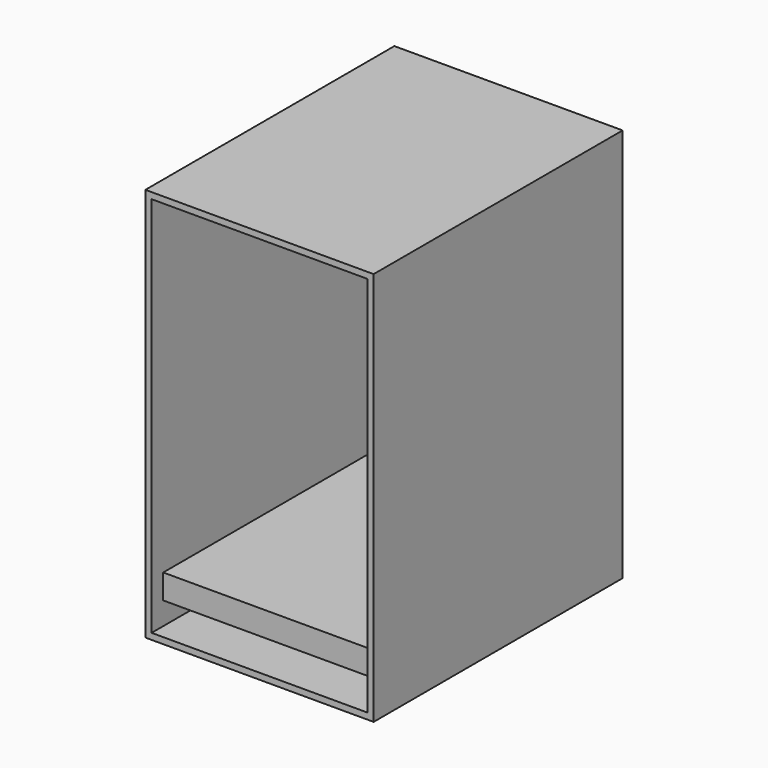
from build123d import *

# Parameters (mm, degrees)
F0_W         = 279.4
F0_H         = 482.6
F1_DEPTH     = 381
F2_T         = -7.62
F3_W         = 264.16
F3_H         = 30.1203280687
F4_DEPTH     = 355.6
F5_W         = 102.4026331621
F5_H         = 105.4210998118
F6_DEPTH     = 177.8
F7_DEPTH     = 177.8
F8_T         = 7.62
F8_T3_DEPTH  = 388.62
F8_T5_DEPTH  = 42.9501895142
F8_T7_DEPTH  = 370.84
F8_T9_DEPTH  = 45.3603280687
F8_T11_DEPTH = 146.3519571328
F8_T13_DEPTH = 193.04
F8_T15_DEPTH = 188.2364254725
F8_T17_DEPTH = 279.4
F8_T19_DEPTH = 424.7694824171
F8_T21_DEPTH = 117.6426331621
F8_T23_DEPTH = 120.6610998118


# Not quite as in the source:
# - a shell that OpenCascade refuses in one call is made with other operations: the cavity is built on its own and cut out


with BuildPart() as f1:
    # F0 (on Front) → F1 (new body)
    with BuildSketch(Plane.XZ):
        Rectangle(F0_W, F0_H)
    extrude(amount=F1_DEPTH)

    # F2
    f2_openings = [f1.faces().sort_by_distance(p)[0] for p in [
        (0, -381, 0),
    ]]
    offset(amount=F2_T, openings=f2_openings)

    # F3 (on face) → F4 (join)
    with BuildSketch(Plane.XZ.offset(7.62)):
        with Locations((0, -190.9096464515)):
            Rectangle(F3_W, F3_H)
    extrude(amount=F4_DEPTH)

    # F5 (on face) → F6 (join)
    with BuildSketch(Plane.XZ.offset(7.62)):
        with Locations((80.8786834189, 7.9730246216)):
            Rectangle(F5_W, F5_H)
    extrude(amount=F6_DEPTH)

    # F7 (add): a face of the model
    f7_faces = [f1.faces().sort_by_distance(p)[0] for p in [
        (80.8786834189, -185.42, 7.9730246216),
    ]]
    extrude(f7_faces, amount=-F7_DEPTH)

    # F8: shell of thickness 7.62, made by hand


with BuildPart() as f8_core1:
    # F8_t2: copy of F1
    add(f1.part)

    # the walls: a layer under each face that stays
    f8_faces = [f8_core1.faces().sort_by_distance(p)[0] for p in [
        (139.7, -190.5, 0),
        (0, -190.5, -241.3),
        (0, -190.5, 241.3),
        (0, 0, 0),
        (96.04375, -381, -235.3419753086),
        (-139.7, -190.5, 0),
        (132.08, -194.31, 0),
        (0, -194.31, -233.68),
        (-132.08, -194.31, 0),
        (0, -194.31, 233.68),
        (0, -7.62, -219.8249052429),
        (0, -185.42, -205.9698104858),
        (0, -363.22, -190.9096464515),
        (0, -185.42, -175.8494824171),
        (0, -7.62, 28.9152587914),
        (80.8786834189, -96.52, -44.7375252843),
        (80.8786834189, -96.52, 60.6835745275),
        (29.6773668379, -96.52, 7.9730246216),
    ]]
    thicken(f8_faces, amount=-F8_T, mode=Mode.SUBTRACT)

    # F8_s4 → F8_t3 (cut)
    with BuildSketch(Plane.XZ):
        Polygon((132.0038, -233.6038), (139.7, -233.68), (139.7, -241.3), (132.08, -241.3), align=None)
        Polygon((132.0038, 233.6038), (139.7, 233.68), (139.7, 241.3), (132.08, 241.3), align=None)
        Polygon((-132.0038, -233.6038), (-132.08, -241.3), (-139.7, -241.3), (-139.7, -233.68), align=None)
        Polygon((-132.0038, 233.6038), (-139.7, 233.68), (-139.7, 241.3), (-132.08, 241.3), align=None)
    extrude(amount=F8_T3_DEPTH, mode=Mode.SUBTRACT)

    # F8_s6 → F8_t5 (cut)
    with BuildSketch(Plane.XY.offset(-241.3)):
        Polygon((132.0038, -7.6962), (139.7, -7.62), (139.7, 0), (132.08, 0), align=None)
        Polygon((-132.0038, -7.6962), (-139.7, -7.62), (-139.7, 0), (-132.08, 0), align=None)
    extrude(amount=F8_T5_DEPTH, mode=Mode.SUBTRACT)

    # F8_s8 → F8_t7 (cut)
    with BuildSketch(Plane.XZ):
        Polygon((132.0038, -206.0460104858), (139.7, -205.9698104858), (139.7, -198.3498104858), (132.08, -198.3498104858), align=None)
        Polygon((132.0038, -175.7732824171), (139.7, -175.8494824171), (139.7, -183.4694824171), (132.08, -183.4694824171), align=None)
        Polygon((-132.0038, -175.7732824171), (-139.7, -175.8494824171), (-139.7, -183.4694824171), (-132.08, -183.4694824171), align=None)
        Polygon((-132.0038, -206.0460104858), (-139.7, -205.9698104858), (-139.7, -198.3498104858), (-132.08, -198.3498104858), align=None)
    extrude(amount=F8_T7_DEPTH, mode=Mode.SUBTRACT)

    # F8_s10 → F8_t9 (cut)
    with BuildSketch(Plane.XY.offset(-213.5898104858)):
        Polygon((132.0038, -363.2962), (139.7, -363.22), (139.7, -355.6), (132.08, -355.6), align=None)
        Polygon((-132.0038, -363.2962), (-139.7, -363.22), (-139.7, -355.6), (-132.08, -355.6), align=None)
    extrude(amount=F8_T9_DEPTH, mode=Mode.SUBTRACT)

    # F8_s12 → F8_t11 (cut)
    with BuildSketch(Plane.XY.offset(-183.4694824171)):
        Polygon((132.0038, -7.6962), (139.7, -7.62), (139.7, 0), (132.08, 0), align=None)
    extrude(amount=F8_T11_DEPTH, mode=Mode.SUBTRACT)

    # F8_s14 → F8_t13 (cut)
    with BuildSketch(Plane.XZ):
        Polygon((132.0038, -44.8137252843), (139.7, -44.7375252843), (139.7, -37.1175252843), (132.08, -37.1175252843), align=None)
        Polygon((132.0038, 60.7597745275), (139.7, 60.6835745275), (139.7, 53.0635745275), (132.08, 53.0635745275), align=None)
    extrude(amount=F8_T13_DEPTH, mode=Mode.SUBTRACT)

    # F8_s16 → F8_t15 (cut)
    with BuildSketch(Plane.XY.offset(53.0635745275)):
        Polygon((132.0038, -7.6962), (139.7, -7.62), (139.7, 0), (132.08, 0), align=None)
    extrude(amount=F8_T15_DEPTH, mode=Mode.SUBTRACT)

    # F8_s18 → F8_t17 (cut)
    with BuildSketch(Plane.YZ.offset(-139.7)):
        Polygon((-7.6962, -233.6038), (-7.62, -241.3), (0, -241.3), (0, -233.68), align=None)
        Polygon((-7.6962, 233.6038), (-7.62, 241.3), (0, 241.3), (0, 233.68), align=None)
        Polygon((-7.6962, -206.0460104858), (0, -205.9698104858), (0, -198.3498104858), (-7.62, -198.3498104858), align=None)
        Polygon((-7.6962, -175.7732824171), (-7.62, -183.4694824171), (0, -183.4694824171), (0, -175.8494824171), align=None)
    extrude(amount=F8_T17_DEPTH, mode=Mode.SUBTRACT)

    # F8_s20 → F8_t19 (cut)
    with BuildSketch(Plane.XY.offset(-183.4694824171)):
        Polygon((-132.0038, -7.6962), (-139.7, -7.62), (-139.7, 0), (-132.08, 0), align=None)
    extrude(amount=F8_T19_DEPTH, mode=Mode.SUBTRACT)

    # F8_s22 → F8_t21 (cut)
    with BuildSketch(Plane.YZ.offset(22.0573668379)):
        Polygon((-7.6962, 60.7597745275), (0, 60.6835745275), (0, 53.0635745275), (-7.62, 53.0635745275), align=None)
        Polygon((-7.6962, -44.8137252843), (0, -44.7375252843), (0, -37.1175252843), (-7.62, -37.1175252843), align=None)
    extrude(amount=F8_T21_DEPTH, mode=Mode.SUBTRACT)

    # F8_s24 → F8_t23 (cut)
    with BuildSketch(Plane.XY.offset(-52.3575252843)):
        Polygon((29.6011668379, -7.6962), (29.6773668379, 0), (37.2973668379, 0), (37.2973668379, -7.62), align=None)
    extrude(amount=F8_T23_DEPTH, mode=Mode.SUBTRACT)


with BuildPart() as f1_1:
    add(f1.part)

    # what is left inside the walls is the cavity
    f8_cavity = [f8_core1.part.solids().sort_by_distance(p)[0] for p in [
        (84.688683, -126.153333, 52.987375),
        (0, -239.606667, -183.545682),
    ]]
    add(f8_cavity, mode=Mode.SUBTRACT)


solid = f1_1.part
